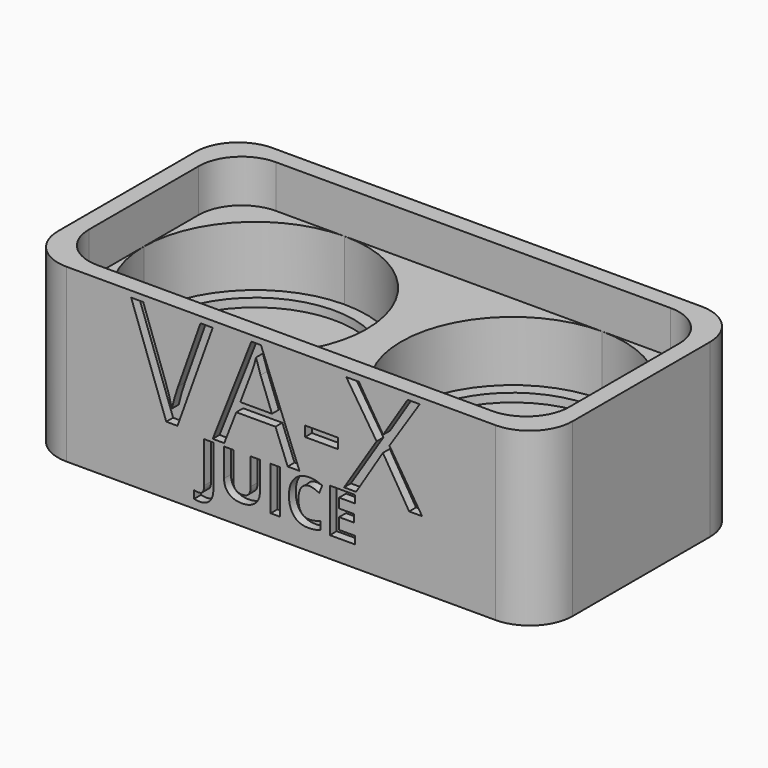
from build123d import *

# Parameters (mm, degrees)
F0_R           = 11.5
F1_DEPTH       = 8
F2_DEPTH       = 15
F3_DEPTH       = 20
F0_R_2         = 4
F4_DEPTH       = 7
F5_TEXT_SIZE   = 15.9761790807
F5_TEXT_SIZE_2 = 7.1291559531
F6_DEPTH       = 1


# Not quite as in the source:
# - Text() gives the source's letters only with a copy of the font that has no kerning and outlines rounded to 1/6400 em; it was checked with that copy


with BuildPart() as f1:
    # F0 (on Top) → F1 (new body)
    with BuildSketch(Plane.XY):
        with BuildLine():
            ThreePointArc((-14.9999999628, -13), (-5.8076118314, -9.1923881423), (-2, 0))
            ThreePointArc((-2, 0), (-5.8076118446, 9.1923881554), (-15, 13))
            ThreePointArc((-15, 13), (-24.1923881554, 9.1923881554), (-28, 0))
            ThreePointArc((-28, 0), (-24.1923881423, -9.1923881686), (-14.9999999628, -13))
        make_face()
        with Locations((-15, 0)):
            Circle(F0_R, mode=Mode.SUBTRACT)
    extrude(amount=F1_DEPTH)


with BuildPart() as f1b:
    # F0 (on Top) → F1, piece 2 (new body)
    with BuildSketch(Plane.XY):
        with BuildLine():
            ThreePointArc((28, 0), (24.1923881554, 9.1923881554), (15, 13))
            ThreePointArc((15, 13), (2, 0), (15, -13))
            ThreePointArc((15, -13), (24.1923881554, -9.1923881554), (28, 0))
        make_face()
        with Locations((15, 0)):
            Circle(F0_R, mode=Mode.SUBTRACT)
    extrude(amount=F1_DEPTH)


with BuildPart() as f2:
    # F0 (on Top) → F2 (new body)
    with BuildSketch(Plane.XY):
        with BuildLine():
            ThreePointArc((-28, 0), (-24.1923881554, 9.1923881554), (-15, 13))
            Line((-15, 13), (-23, 13))
            ThreePointArc((-23, 13), (-26.5355339059, 11.5355339059), (-28, 8))
            Line((-28, 8), (-28, 0))
        make_face()
    extrude(amount=F2_DEPTH)


with BuildPart() as f2b:
    # F0 (on Top) → F2, piece 2 (new body)
    with BuildSketch(Plane.XY):
        with BuildLine():
            Line((-23, -13), (-14.9999999628, -13))
            ThreePointArc((-14.9999999628, -13), (-24.1923881423, -9.1923881686), (-28, 0))
            Line((-28, 0), (-28, -8))
            ThreePointArc((-28, -8), (-26.5355339059, -11.5355339059), (-23, -13))
        make_face()
    extrude(amount=F2_DEPTH)


with BuildPart() as f2c:
    # F0 (on Top) → F2, piece 3 (new body)
    with BuildSketch(Plane.XY):
        with BuildLine():
            ThreePointArc((-15, 13), (-5.8076118446, 9.1923881554), (-2, 0))
            ThreePointArc((-2, 0), (-5.8076118314, -9.1923881423), (-14.9999999628, -13))
            Line((-14.9999999628, -13), (15, -13))
            ThreePointArc((15, -13), (2, 0), (15, 13))
            Line((15, 13), (-15, 13))
        make_face()
    extrude(amount=F2_DEPTH)

    # F0 (on Top) → F3 (join)
    with BuildSketch(Plane.XY):
        with BuildLine():
            ThreePointArc((30, 10), (28.5355339059, 13.5355339059), (25, 15))
            Line((25, 15), (-25, 15))
            ThreePointArc((-25, 15), (-28.5355339059, 13.5355339059), (-30, 10))
            Line((-30, 10), (-30, -10))
            ThreePointArc((-30, -10), (-28.5355339059, -13.5355339059), (-25, -15))
            Line((-25, -15), (25, -15))
            ThreePointArc((25, -15), (28.5355339059, -13.5355339059), (30, -10))
            Line((30, -10), (30, 10))
        make_face()
        with BuildLine():
            Line((-23, 13), (-15, 13))
            Line((-15, 13), (15, 13))
            Line((15, 13), (23, 13))
            ThreePointArc((23, 13), (26.5355339059, 11.5355339059), (28, 8))
            Line((28, 8), (28, 0))
            Line((28, 0), (28, -8))
            ThreePointArc((28, -8), (26.5355339059, -11.5355339059), (23, -13))
            Line((23, -13), (15, -13))
            Line((15, -13), (-14.9999999628, -13))
            Line((-14.9999999628, -13), (-23, -13))
            ThreePointArc((-23, -13), (-26.5355339059, -11.5355339059), (-28, -8))
            Line((-28, -8), (-28, 0))
            Line((-28, 0), (-28, 8))
            ThreePointArc((-28, 8), (-26.5355339059, 11.5355339059), (-23, 13))
        make_face(mode=Mode.SUBTRACT)
    extrude(amount=F3_DEPTH)

    # F5 (on face) → F6 (cut)
    with BuildSketch(Plane.XZ.offset(15)):
        with Locations((-17.4764421475, 7.8760646284)):
            Text('VA-X', F5_TEXT_SIZE, font='Open Sans', text_align=(TextAlign.LEFT, TextAlign.BOTTOM))
        with Locations((-9.6076515774, 2.4338566)):
            Text('JUICE', F5_TEXT_SIZE_2, font='Open Sans', font_style=FontStyle.BOLD, text_align=(TextAlign.LEFT, TextAlign.BOTTOM))
    extrude(amount=-F6_DEPTH, mode=Mode.SUBTRACT)


with BuildPart() as f2d:
    # F0 (on Top) → F2, piece 4 (new body)
    with BuildSketch(Plane.XY):
        with BuildLine():
            Line((23, 13), (15, 13))
            ThreePointArc((15, 13), (24.1923881554, 9.1923881554), (28, 0))
            Line((28, 0), (28, 8))
            ThreePointArc((28, 8), (26.5355339059, 11.5355339059), (23, 13))
        make_face()
    extrude(amount=F2_DEPTH)


with BuildPart() as f2e:
    # F0 (on Top) → F2, piece 5 (new body)
    with BuildSketch(Plane.XY):
        with BuildLine():
            ThreePointArc((28, 0), (24.1923881554, -9.1923881554), (15, -13))
            Line((15, -13), (23, -13))
            ThreePointArc((23, -13), (26.5355339059, -11.5355339059), (28, -8))
            Line((28, -8), (28, 0))
        make_face()
    extrude(amount=F2_DEPTH)


with BuildPart() as f4:
    # F0 (on Top) → F4 (new body)
    with BuildSketch(Plane.XY):
        with Locations((-15, 0)):
            Circle(F0_R)
        with Locations((-15, 0)):
            Circle(F0_R_2, mode=Mode.SUBTRACT)
    extrude(amount=F4_DEPTH)


with BuildPart() as f4b:
    # F0 (on Top) → F4, piece 2 (new body)
    with BuildSketch(Plane.XY):
        with Locations((15, 0)):
            Circle(F0_R)
        with Locations((15, 0)):
            Circle(F0_R_2, mode=Mode.SUBTRACT)
    extrude(amount=F4_DEPTH)


solid = Compound([f1.part, f1b.part, f2.part, f2b.part, f2c.part, f2d.part, f2e.part, f4.part, f4b.part])
